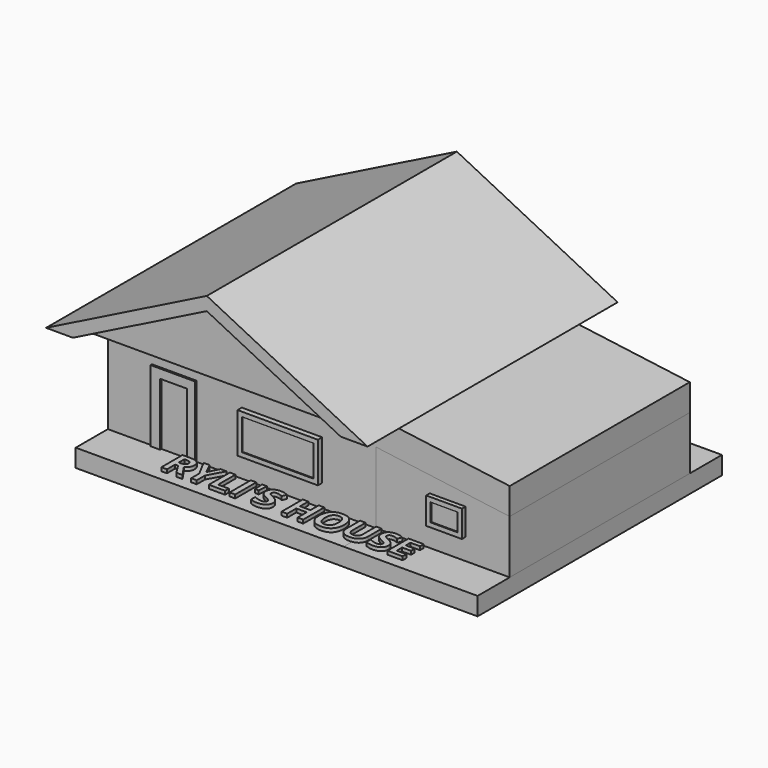
from build123d import *

# Parameters (mm, degrees)
F1_DEPTH      = 5334
F2_DEPTH      = 4815.84
F3_DEPTH      = 5212.08
F0_W          = 2743.2
F0_H          = 1371.6
F4_DEPTH      = 3840.48
F5_DEPTH      = 3840.48
F6_DEPTH      = 3901.44
F0_W_2        = 2438.4
F0_H_2        = 1066.8
F7_DEPTH      = 4023.36
F0_W_3        = 1219.2
F0_H_3        = 914.4
F8_DEPTH      = 3840.48
F9_DEPTH      = 3992.88
F0_W_4        = 914.4
F0_H_4        = 2133.6
F10_DEPTH     = 3840.48
F0_H_5        = 609.6
F11_DEPTH     = 3992.88
F12_DEPTH     = 3962.4
F13_TEXT_SIZE = 1259.6415148841
F14_DEPTH     = 121.92


# Not quite as in the source:
# - Text() gives the source's letters only with a copy of the font that has no kerning and outlines rounded to 1/6400 em; it was checked with that copy


with BuildPart() as f1:
    # F0 (on Front) → F1 (new body, symmetric)
    with BuildSketch(Plane.XZ):
        Polygon((4572, 6096), (4572, 5638.8), (9144, 3352.8), (10058.5058323126, 3352.7470838437), align=None)
        Polygon((-914.4, 3352.8), (0, 3352.8), (4572, 5638.8), (4572, 6096), align=None)
    extrude(amount=F1_DEPTH, both=True)

    # F0 (on Front) → F2 (join, symmetric)
    with BuildSketch(Plane.XZ):
        Polygon((4572, 5638.8), (0, 3352.8), (4572, 3352.8), align=None)
        Polygon((4572, 5638.8), (4572, 3352.8), (9144, 3352.8), align=None)
    extrude(amount=F2_DEPTH, both=True)


with BuildPart() as f3:
    # F0 (on Front) → F3 (new body, symmetric)
    with BuildSketch(Plane.XZ):
        Polygon((9144, 0), (9144, -609.6), (13715.9956149355, -609.6), (13715.9956149355, 6.33222), align=None)
        Polygon((1506.0168, 0), (0, 0), (0, -609.6), (9144, -609.6), (9144, 0), (4572, 0), (3030.0168, 0), (2743.2, 0), (1828.8, 0), align=None)
    extrude(amount=F3_DEPTH, both=True)

    # F13 (on face) → F14 (join, symmetric)
    with BuildSketch(Plane.XY):
        with Locations((2520.6019878387, -4849.0619659424)):
            Text("RYLI'S HOUSE", F13_TEXT_SIZE, font='Open Sans', font_style=FontStyle.BOLD, text_align=(TextAlign.LEFT, TextAlign.BOTTOM))
    extrude(amount=F14_DEPTH, both=True)


with BuildPart() as f4:
    # F0 (on Front) → F4 (new body, symmetric)
    with BuildSketch(Plane.XZ):
        Polygon((0, 3352.8), (0, 0), (1506.0168, 0), (1506.0168, 2438.4), (3030.0168, 2438.4), (3030.0168, 0), (4572, 0), (9144, 0), (9144, 2438.4), (9144, 3352.8), (4572, 3352.8), align=None)
        with Locations((5943.6, 1447.8)):
            Rectangle(F0_W, F0_H, mode=Mode.SUBTRACT)
    extrude(amount=F4_DEPTH, both=True)

    # F0 (on Front) → F5 (join, symmetric)
    with BuildSketch(Plane.XZ):
        Polygon((13715.9956149355, 2749.53222), (9144, 3352.8), (9144, 2438.4), (13715.9956149355, 1835.13222), align=None)
    extrude(amount=F5_DEPTH, both=True)

    # F0 (on Front) → F7 (join, symmetric)
    with BuildSketch(Plane.XZ):
        with Locations((5943.6, 1447.8)):
            Rectangle(F0_W, F0_H)
        with Locations((5943.6, 1447.8)):
            Rectangle(F0_W_2, F0_H_2, mode=Mode.SUBTRACT)
    extrude(amount=F7_DEPTH, both=True)


with BuildPart() as f6:
    # F0 (on Front) → F6 (new body, symmetric)
    with BuildSketch(Plane.XZ):
        Polygon((1506.0168, 2438.4), (1506.0168, 0), (1828.8, 0), (1828.8, 2133.6), (2743.2, 2133.6), (2743.2, 0), (3030.0168, 0), (3030.0168, 2438.4), align=None)
    extrude(amount=F6_DEPTH, both=True)


with BuildPart() as f8:
    # F0 (on Front) → F8 (new body, symmetric)
    with BuildSketch(Plane.XZ):
        Polygon((9144, 2438.4), (9144, 0), (13715.9956149355, 6.33222), (13715.9956149355, 1835.13222), align=None)
        with Locations((11595.2576919556, 1184.6426817894)):
            Rectangle(F0_W_3, F0_H_3, mode=Mode.SUBTRACT)
    extrude(amount=F8_DEPTH, both=True)


with BuildPart() as f9:
    # F0 (on Front) → F9 (new body, symmetric)
    with BuildSketch(Plane.XZ):
        with Locations((5943.6, 1447.8)):
            Rectangle(F0_W_2, F0_H_2)
    extrude(amount=F9_DEPTH, both=True)


with BuildPart() as f10:
    # F0 (on Front) → F10 (new body, symmetric)
    with BuildSketch(Plane.XZ):
        with Locations((2286, 1066.8)):
            Rectangle(F0_W_4, F0_H_4)
    extrude(amount=F10_DEPTH, both=True)


with BuildPart() as f11:
    # F0 (on Front) → F11 (new body, symmetric)
    with BuildSketch(Plane.XZ):
        with Locations((11595.2576919556, 1184.6426817894)):
            Rectangle(F0_W_3, F0_H_3)
        with Locations((11595.2576919556, 1184.6426817894)):
            Rectangle(F0_W_4, F0_H_5, mode=Mode.SUBTRACT)
    extrude(amount=F11_DEPTH, both=True)


with BuildPart() as f12:
    # F0 (on Front) → F12 (new body, symmetric)
    with BuildSketch(Plane.XZ):
        with Locations((11595.2576919556, 1184.6426817894)):
            Rectangle(F0_W_4, F0_H_5)
    extrude(amount=F12_DEPTH, both=True)


solid = Compound([f1.part, f3.part, f4.part, f6.part, f8.part, f9.part, f10.part, f11.part, f12.part])
